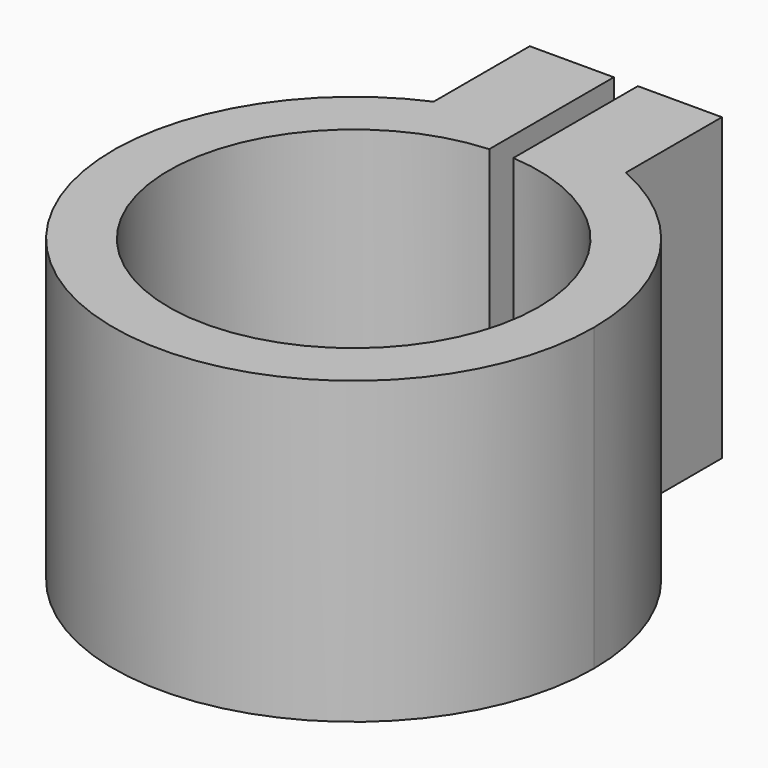
from build123d import *

# Parameters (mm, degrees)
F1_DEPTH = 25


# Not quite as in the source:
# - a feature names something its author has since deleted; it is built from what else it names


with BuildPart() as f1:
    # F0 (on Top) → F1 (new body)
    with BuildSketch(Plane.XY):
        with BuildLine():
            ThreePointArc((1, 15.3674981698), (11.2374374303, 10.5299572649), (15.4, 0))
            ThreePointArc((15.4, 0), (-10.5299572649, -11.2374374303), (-1, 15.3674981698))
            Line((-1, 15.3674981698), (-1, 19.9749843554))
            ThreePointArc((-1, 19.9749843554), (-4.5745212177, 19.4698165279), (-8, 18.3303027798))
            ThreePointArc((-8, 18.3303027798), (-10.9544511501, -16.7332005307), (20, 0))
            ThreePointArc((20, 0), (16.7332005307, 10.9544511501), (8, 18.3303027798))
            ThreePointArc((8, 18.3303027798), (4.5745212177, 19.4698165279), (1, 19.9749843554))
            Line((1, 19.9749843554), (1, 15.3674981698))
        make_face()
        with BuildLine():
            Line((1, 28.3303027798), (1, 19.9749843554))
            ThreePointArc((1, 19.9749843554), (4.5745212177, 19.4698165279), (8, 18.3303027798))
            Line((8, 18.3303027798), (8, 28.3303027798))
            Line((8, 28.3303027798), (1, 28.3303027798))
        make_face()
        with BuildLine():
            ThreePointArc((-8, 18.3303027798), (-4.5745212177, 19.4698165279), (-1, 19.9749843554))
            Line((-1, 19.9749843554), (-1, 28.3303027798))
            Line((-1, 28.3303027798), (-8, 28.3303027798))
            Line((-8, 28.3303027798), (-8, 18.3303027798))
        make_face()
    extrude(amount=F1_DEPTH)


solid = f1.part
